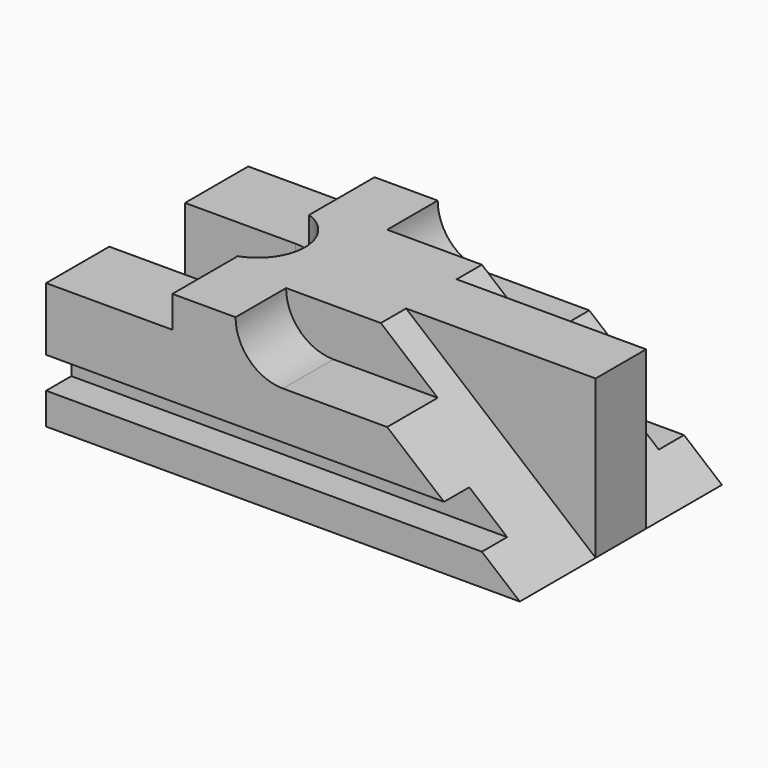
from build123d import *

# Parameters (mm, degrees)
F1_DEPTH = 50
F2_W     = 40
F2_H     = 10
F3_DEPTH = 30
F4_DEPTH = 10
F5_DEPTH = 20


# Not quite as in the source:
# - a pattern or mirror of a feature is missing from the dataset's text; its kind, count and spacing are read off the source's solid


with BuildPart() as f1:
    # F0 (on Top) → F1 (new body)
    with BuildSketch(Plane.XY):
        with BuildLine():
            Line((-35, -15), (-35, -40))
            Line((-35, -40), (115, -40))
            Line((115, -40), (115, 40))
            Line((115, 40), (-35, 40))
            Line((-35, 40), (-35, 15))
            Line((-35, 15), (0, 15))
            ThreePointArc((0, 15), (15, 0), (0, -15))
            Line((0, -15), (-35, -15))
        make_face()
    extrude(amount=F1_DEPTH)

    # F2 (on face) → F3 (cut)
    with BuildSketch(Plane.XZ.offset(40)):
        with Locations((-15, 45)):
            Rectangle(F2_W, F2_H)
        Polygon((115, 50), (55, 50), (73, 35), (91, 20), (103, 10), (115, 0), align=None)
    f3 = extrude(amount=-F3_DEPTH, mode=Mode.SUBTRACT)

    # F3_copies: F3 across plane
    add(f3.mirror(Plane.ZX), mode=Mode.SUBTRACT)

    # F2 (on face) → F4 (cut)
    with BuildSketch(Plane.XZ.offset(40)):
        Polygon((91, 20), (-35, 20), (-35, 10), (103, 10), align=None)
    f4 = extrude(amount=-F4_DEPTH, mode=Mode.SUBTRACT)

    # F4_copies: F4 across plane
    add(f4.mirror(Plane.ZX), mode=Mode.SUBTRACT)

    # F2 (on face) → F5 (cut)
    with BuildSketch(Plane.XZ.offset(40)):
        with BuildLine():
            Line((55, 50), (25, 50))
            ThreePointArc((25, 50), (29.3933982822, 39.3933982822), (40, 35))
            Line((40, 35), (73, 35))
            Line((73, 35), (55, 50))
        make_face()
    f5 = extrude(amount=-F5_DEPTH, mode=Mode.SUBTRACT)

    # F5_copies: F5 across plane
    add(f5.mirror(Plane.ZX), mode=Mode.SUBTRACT)


solid = f1.part
